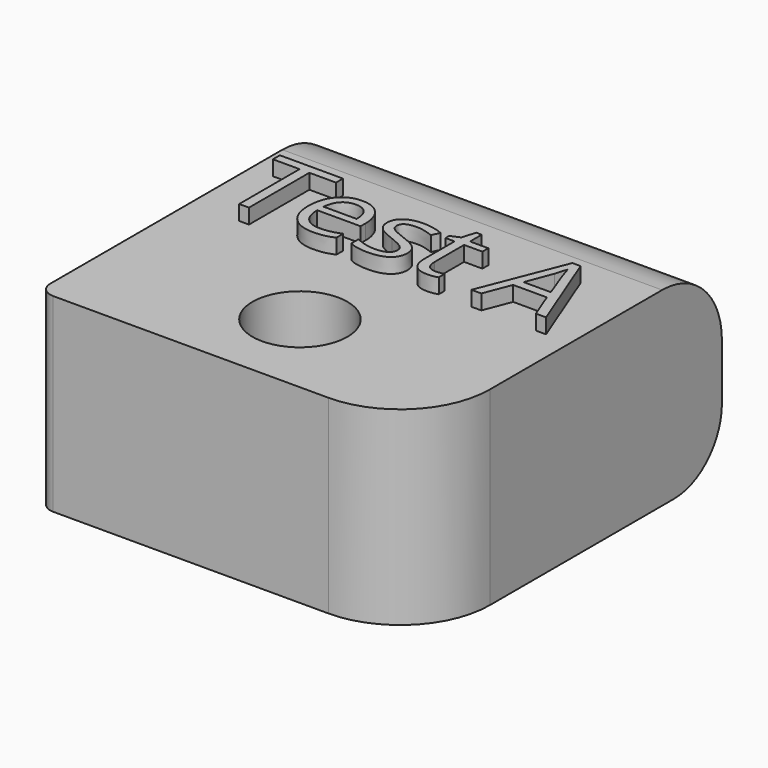
from build123d import *

# Parameters (mm, degrees)
F0_W         = 25.4
F0_H         = 25.4
F1_DEPTH     = 12.7
F2_R         = 3.175
F3_DEPTH     = 12.701
F4_R         = 6
F5_R         = 1
F6_R         = 5
F7_R         = 4
F8_TEXT_SIZE = 7.8871225317
F9_DEPTH     = 1


# Not quite as in the source:
# - Text() gives the source's letters only with a copy of the font that has no kerning and outlines rounded to 1/6400 em; it was checked with that copy


with BuildPart() as f1:
    # F0 (on Top) → F1 (new body)
    with BuildSketch(Plane.XY):
        Rectangle(F0_W, F0_H)
    extrude(amount=F1_DEPTH)

    # F2 (on face) → F3 (cut, through all)
    with BuildSketch(Plane.XY.offset(12.7)):
        with Locations((0, -6.7)):
            Circle(F2_R)
    extrude(amount=-F3_DEPTH, mode=Mode.SUBTRACT)

    # F4
    f4_edges = [f1.edges().sort_by_distance(p)[0] for p in [
        (12.7, -12.7, 6.35),
    ]]
    fillet(f4_edges, radius=F4_R)

    # F5
    f5_edges = [f1.edges().sort_by_distance(p)[0] for p in [
        (-12.7, -12.7, 6.35),
    ]]
    fillet(f5_edges, radius=F5_R)

    # F6
    f6_edges = [f1.edges().sort_by_distance(p)[0] for p in [
        (0, 12.7, 12.7),
    ]]
    fillet(f6_edges, radius=F6_R)

    # F7
    f7_edges = [f1.edges().sort_by_distance(p)[0] for p in [
        (0, 12.7, 0),
    ]]
    fillet(f7_edges, radius=F7_R)

    # F8 (on face) → F9 (join)
    with BuildSketch(Plane.XY.offset(12.7)):
        with Locations((-11.277503334, 0)):
            Text('Test A', F8_TEXT_SIZE, font='Open Sans', text_align=(TextAlign.LEFT, TextAlign.BOTTOM))
    extrude(amount=F9_DEPTH)


solid = f1.part
